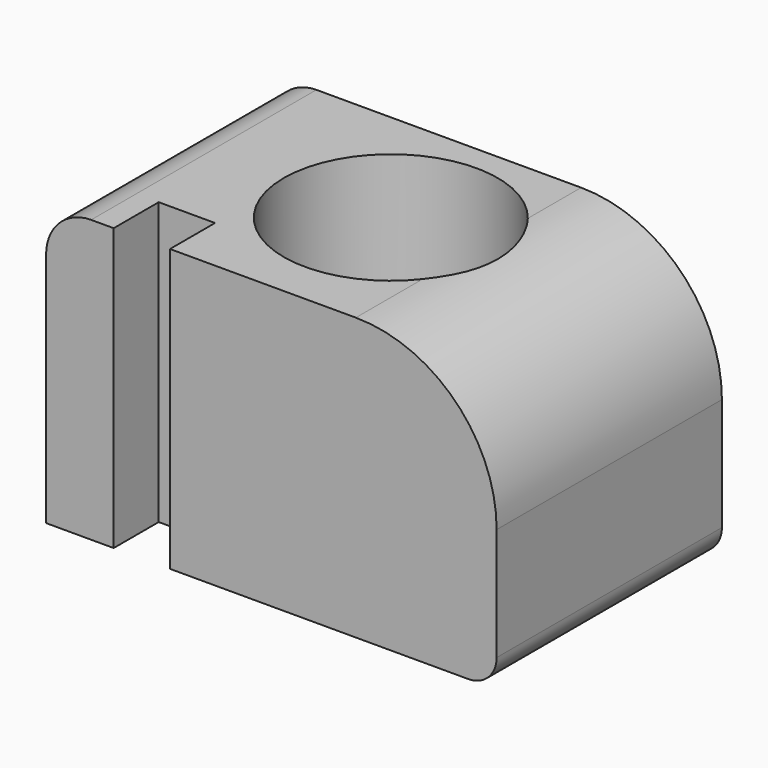
from build123d import *

# Parameters (mm, degrees)
F0_W        = 80
F0_H        = 50
F0_R        = 19
F1_DEPTH    = 50
F2_T1_DEPTH = 175
F3_R        = 5
F4_R        = 8
F5_W        = 10
F5_H        = 50
F6_DEPTH    = 10


# Not quite as in the source:
# - a fillet or chamfer that OpenCascade refuses, or shapes differently, is made with other operations: its cross-section is extruded or revolved along the edge and cut away or added


with BuildPart() as f1:
    # F0 (on Top) → F1 (new body)
    with BuildSketch(Plane.XY):
        with Locations((0, -1.5042735598)):
            Rectangle(F0_W, F0_H)
        Circle(F0_R, mode=Mode.SUBTRACT)
    extrude(amount=-F1_DEPTH)

    # F2: fillet of radius 25 on 1 edges, made by hand

    # F2_s2 → F2_t1 (cut)
    with BuildSketch(Plane.XZ.offset(-85.9957264402)):
        with BuildLine():
            ThreePointArc((40, -25), (32.6776695297, -7.3223304703), (15, 0))
            Line((15, 0), (40, 0))
            Line((40, 0), (40, -25))
        make_face()
    extrude(amount=F2_T1_DEPTH, mode=Mode.SUBTRACT)

    # F3
    f3_edges = [f1.edges().sort_by_distance(p)[0] for p in [
        (40, -1.504274, -50),
    ]]
    fillet(f3_edges, radius=F3_R)

    # F4
    f4_edges = [f1.edges().sort_by_distance(p)[0] for p in [
        (-40, -1.504274, 0),
    ]]
    fillet(f4_edges, radius=F4_R)

    # F5 (on face) → F6 (cut)
    with BuildSketch(Plane.XZ.offset(26.5042735598)):
        with Locations((-23, -25)):
            Rectangle(F5_W, F5_H)
    extrude(amount=-F6_DEPTH, mode=Mode.SUBTRACT)


solid = f1.part
